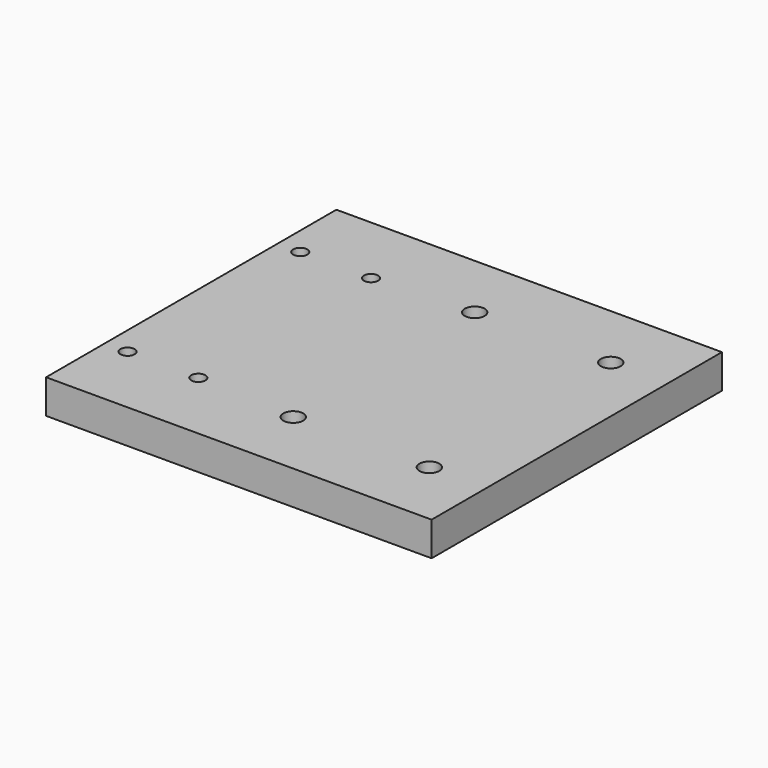
from build123d import *

# Parameters (mm, degrees)
F0_W     = 215.9
F0_H     = 203.2
F1_DEPTH = 19.05
F3_D     = 11.1125
F5_D     = 7.9375


# Not quite as in the source:
# - a length typed as a fraction of an inch, garbled in the dataset ("3 / 203.2 mm" for 3/8 in), is restored


with BuildPart() as f1:
    # F0 (on Top) → F1 (new body)
    with BuildSketch(Plane.XY):
        Rectangle(F0_W, F0_H)
    extrude(amount=F1_DEPTH)

    # F3 (through all)
    with Locations(Plane.XY.offset(19.05)):
        with Locations((0, -63.5), (76.2, -63.5), (76.2, 63.5), (0, 63.5)):
            Hole(F3_D / 2)

    # F5 (through all)
    with Locations(Plane.XY.offset(19.05)):
        with Locations((-95.25, 60.452), (-55.626, 60.452), (-95.25, -60.452), (-55.626, -60.452)):
            Hole(F5_D / 2)


solid = f1.part
